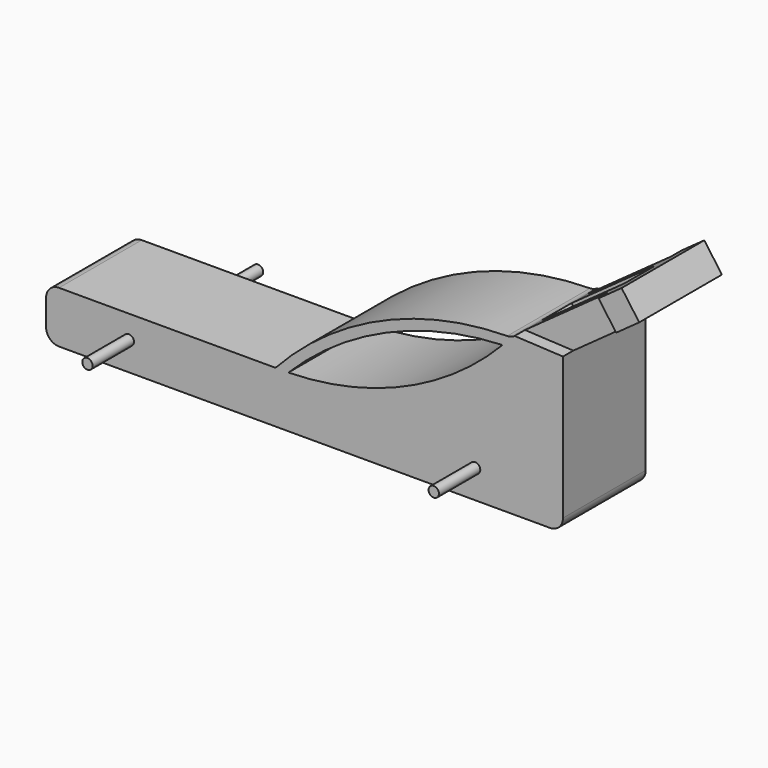
from build123d import *

# Parameters (mm, degrees)
F1_DEPTH  = 40
F2_R      = 5
F7_DEPTH  = 5
F9_DEPTH  = 5
F10_W     = 40
F10_H     = 15
F11_DEPTH = 11.684
F3_R      = 2
F12_DEPTH = 20
F4_R      = 2
F13_DEPTH = 20


# Not quite as in the source:
# - two fillets or chamfers of one size are made in one step


with BuildPart() as f1:
    # F0 (on Front) → F1 (new body)
    with BuildSketch(Plane.XZ):
        with BuildLine():
            Line((0, 20), (0, 0))
            Line((0, 0), (200, 0))
            Line((200, 0), (200, 60))
            Line((200, 60), (180, 60))
            ThreePointArc((180, 60), (178.3255687097, 58.1433963871), (176.6122992708, 56.3225710381))
            ThreePointArc((176.6122992708, 56.3225710381), (138.7955155822, 29.9352120782), (93.7655988336, 20))
            ThreePointArc((93.7655988336, 20), (91.2655988336, 19.9735969417), (88.7655988336, 20))
            Line((88.7655988336, 20), (0, 20))
        make_face()
        with BuildLine():
            ThreePointArc((180, 60), (130.1910752068, 49.5607362037), (88.7655988336, 20))
            ThreePointArc((88.7655988336, 20), (91.2655988336, 19.9735969417), (93.7655988336, 20))
            ThreePointArc((93.7655988336, 20), (131.7599412204, 45.9823724222), (176.6122992708, 56.3225710381))
            ThreePointArc((176.6122992708, 56.3225710381), (178.3255687097, 58.1433963871), (180, 60))
        make_face()
        Polygon((180, 60), (200, 60), (229.4970817654, 81.2315874186), (222.6715144816, 90.714360058), align=None)
    extrude(amount=F1_DEPTH)

    # F2
    f2_edges = [f1.edges().sort_by_distance(p)[0] for p in [
        (0, -20, 20),
        (0, -20, 0),
        (200, -20, 0),
        (180, -20, 60),
    ]]
    fillet(f2_edges, radius=F2_R)

    # F6 (on face) → F7 (cut)
    with BuildSketch(Plane.XZ.offset(40)):
        Polygon((181.2943636671, 60.931664887), (200, 60), (220.5845981647, 74.8165062187), (213.7590308809, 84.2992788581), align=None)
    extrude(amount=-F7_DEPTH, mode=Mode.SUBTRACT)

    # F8 (on face) → F9 (cut)
    with BuildSketch(Plane(origin=(0, 0, 0), x_dir=(-1, 0, 0), z_dir=(0, 1, 0))):
        Polygon((-220.5845981647, 74.8165062187), (-200, 60), (-181.2943636671, 60.931664887), (-213.7590308809, 84.2992788581), align=None)
    extrude(amount=-F9_DEPTH, mode=Mode.SUBTRACT)

    # F10 (on face) → F11 (cut)
    with BuildSketch(Plane(origin=(32.9817876356, 0, -45.8216556055), x_dir=(0.8116166803, 0, 0.5841903493), z_dir=(-0.5841903493, 0, 0.8116166803))):
        with Locations((202.737220197, -20)):
            Rectangle(F10_W, F10_H)
    extrude(amount=-F11_DEPTH, mode=Mode.SUBTRACT)

    # F3 (on face) → F12 (join)
    with BuildSketch(Plane.XZ.offset(40)):
        with Locations((32, 11)):
            Circle(F3_R)
        with Locations((166, 11)):
            Circle(F3_R)
    extrude(amount=F12_DEPTH)

    # F4 (on face) → F13 (join)
    with BuildSketch(Plane(origin=(0, 0, 0), x_dir=(-1, 0, 0), z_dir=(0, 1, 0))):
        with Locations((-166, 11)):
            Circle(F4_R)
        with Locations((-34, 11)):
            Circle(F4_R)
    extrude(amount=F13_DEPTH)


solid = f1.part
